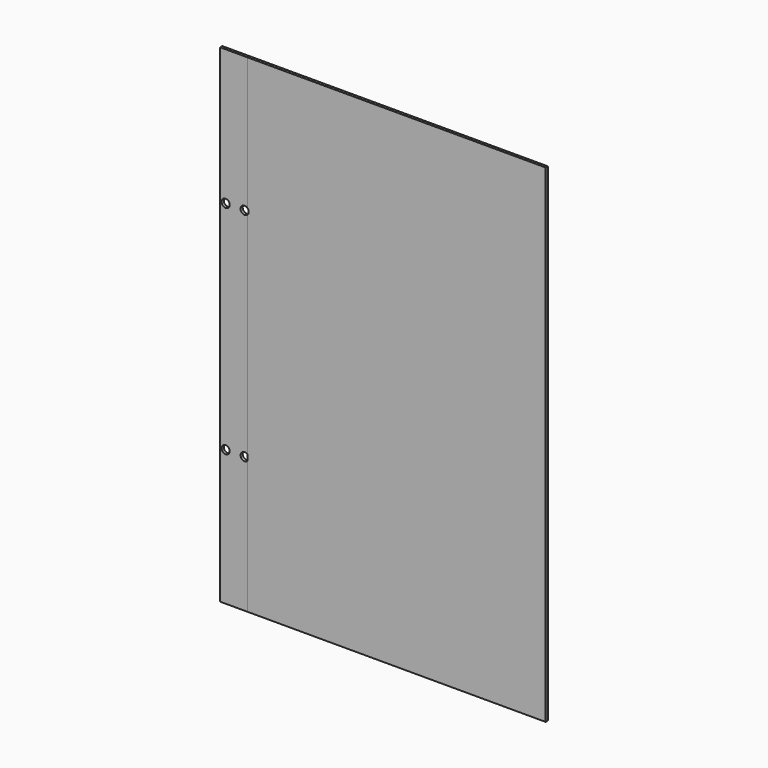
from build123d import *

# Parameters (mm, degrees)
F1_DEPTH = 90
F2_DEPTH = 90
F3_R     = 1.5
F4_DEPTH = 12.5


# Not quite as in the source:
# - a pattern or mirror of a feature is missing from the dataset's text; its kind, count and spacing are read off the source's solid


with BuildPart() as f1:
    # F0 (on Top) → F1 (new body, symmetric)
    with BuildSketch(Plane.XY):
        Polygon((10, 0.5), (0, 0.5), (0, -0.5), (10, -0.5), (120, -0.05), (120, 0.05), align=None)
    extrude(amount=F1_DEPTH, both=True)


with BuildPart() as f2:
    # F0 (on Top) → F2 (new body, symmetric)
    with BuildSketch(Plane.XY):
        Polygon((120, 0.5), (10, 0.5), (120, 0.05), align=None)
    extrude(amount=F2_DEPTH, both=True)


with BuildPart() as f2b:
    # F0 (on Top) → F2, piece 2 (new body, symmetric)
    with BuildSketch(Plane.XY):
        Polygon((120, -0.05), (10, -0.5), (120, -0.5), align=None)
    extrude(amount=F2_DEPTH, both=True)


with BuildPart() as f4_tool:
    # F3 (on Front) → F4 (new body, symmetric)
    with BuildSketch(Plane.XZ):
        with Locations((2, 40)):
            Circle(F3_R)
        with Locations((9, 40)):
            Circle(F3_R)
    f4 = extrude(amount=F4_DEPTH, both=True)


with BuildPart() as f1_1:
    add(f1.part)

    # F4: cut by f4_tool
    add(f4_tool.part, mode=Mode.SUBTRACT)

    # F4_copies: F4 across plane
    add(f4.mirror(Plane(origin=(0, 0, 0), x_dir=(-1, 0, 0), z_dir=(0, 0, -1))), mode=Mode.SUBTRACT)


with BuildPart() as f2_1:
    add(f2.part)

    # F4: cut by f4_tool
    add(f4_tool.part, mode=Mode.SUBTRACT)


with BuildPart() as f2b_1:
    add(f2b.part)

    # F4: cut by f4_tool
    add(f4_tool.part, mode=Mode.SUBTRACT)


solid = Compound([f1_1.part, f2_1.part, f2b_1.part])
